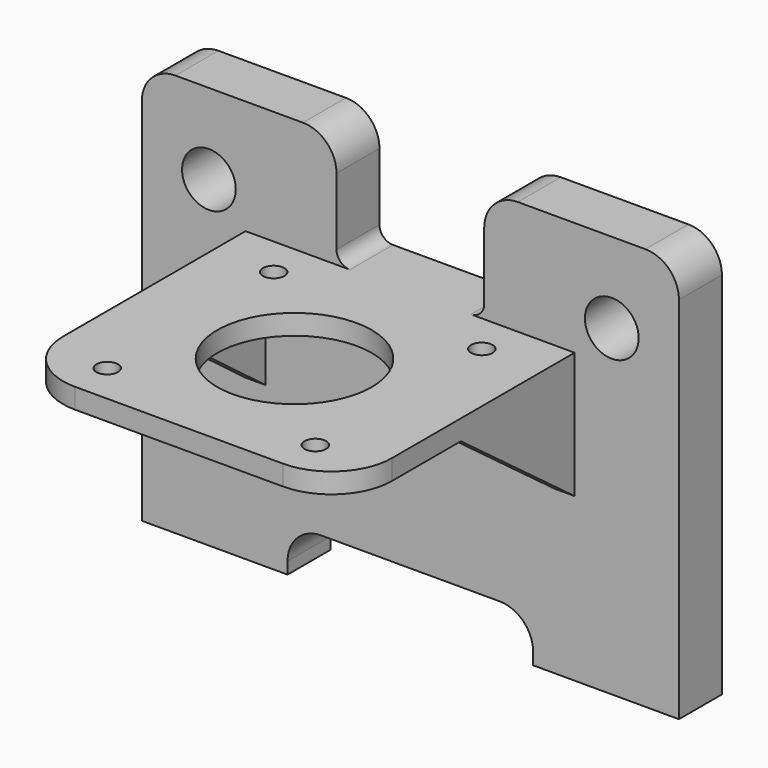
from build123d import *

# Parameters (mm, degrees)
F0_R     = 5
F0_R_2   = 4
F1_DEPTH = 8
F2_W     = 49
F2_H     = 43
F2_R     = 1.6
F2_R_2   = 11.5
F3_DEPTH = 3
F5_DEPTH = 3
F6_R     = 9
F8_DEPTH = 3
F9_DEPTH = 8


# Not quite as in the source:
# - a feature of the source that left no trace in its solid (it failed there, or was rolled back) is left out


with BuildPart() as f1:
    # F0 (on Front) → F1 (new body)
    with BuildSketch(Plane.XZ):
        with BuildLine():
            Line((-15.9509392173, 58.3590910856), (-34.9509392173, 58.3590910856))
            ThreePointArc((-34.9509392173, 58.3590910856), (-38.4864731233, 56.8946249915), (-39.9509392173, 53.3590910856))
            Line((-39.9509392173, 53.3590910856), (-39.9509392173, -1.6409089144))
            Line((-39.9509392173, -1.6409089144), (-18.2393845171, -1.6409089144))
            Line((-18.2393845171, -1.6409089144), (-18.2393845171, 0.1278397727))
            ThreePointArc((-18.2393845171, 0.1278397727), (-16.774918423, 3.6633736787), (-13.2393845171, 5.1278397727))
            Line((-13.2393845171, 5.1278397727), (13.3375060824, 5.1278397727))
            ThreePointArc((13.3375060824, 5.1278397727), (16.8730399883, 3.6633736787), (18.3375060824, 0.1278397727))
            Line((18.3375060824, 0.1278397727), (18.3375060824, -1.6409089144))
            Line((18.3375060824, -1.6409089144), (40.0490607827, -1.6409089144))
            Line((40.0490607827, -1.6409089144), (40.0490607827, 53.3590910856))
            ThreePointArc((40.0490607827, 53.3590910856), (38.5845946886, 56.8946249915), (35.0490607827, 58.3590910856))
            Line((35.0490607827, 58.3590910856), (16.0490607827, 58.3590910856))
            ThreePointArc((16.0490607827, 58.3590910856), (12.5135268767, 56.8946249915), (11.0490607827, 53.3590910856))
            Line((11.0490607827, 53.3590910856), (11.0490607827, 43.3590910856))
            ThreePointArc((11.0490607827, 43.3590910856), (10.463274345, 41.9448775232), (9.0490607827, 41.3590910856))
            Line((9.0490607827, 41.3590910856), (-8.9509392173, 41.3590910856))
            ThreePointArc((-8.9509392173, 41.3590910856), (-10.3651527797, 41.9448775232), (-10.9509392173, 43.3590910856))
            Line((-10.9509392173, 43.3590910856), (-10.9509392173, 53.3590910856))
            ThreePointArc((-10.9509392173, 53.3590910856), (-12.4154053114, 56.8946249915), (-15.9509392173, 58.3590910856))
        make_face()
        with Locations((-29.9509392173, 10.3590910856)):
            Circle(F0_R, mode=Mode.SUBTRACT)
        with Locations((30.0490607827, 10.3590910856)):
            Circle(F0_R, mode=Mode.SUBTRACT)
        with Locations((-29.9509392173, 46.3590910856)):
            Circle(F0_R_2, mode=Mode.SUBTRACT)
        with Locations((30.0490607827, 46.3590910856)):
            Circle(F0_R_2, mode=Mode.SUBTRACT)
    extrude(amount=F1_DEPTH)

    # F2 (on face) → F3 (join)
    with BuildSketch(Plane.XY.offset(41.3590910856)):
        with Locations((0.0111820996, -29.5)):
            Rectangle(F2_W, F2_H)
        with Locations((-15.5, -45)):
            Circle(F2_R, mode=Mode.SUBTRACT)
        with Locations((15.5, -45)):
            Circle(F2_R, mode=Mode.SUBTRACT)
        with Locations((0, -29.5)):
            Circle(F2_R_2, mode=Mode.SUBTRACT)
        with Locations((-15.5, -14)):
            Circle(F2_R, mode=Mode.SUBTRACT)
        with Locations((15.5, -14)):
            Circle(F2_R, mode=Mode.SUBTRACT)
    extrude(amount=-F3_DEPTH)

    # F4 (on face) → F5 (join)
    with BuildSketch(Plane(origin=(-24.4888179004, 0, 0), x_dir=(0, -1, 0), z_dir=(-1, 0, 0))):
        Polygon((29.5, 38.3590910856), (8, 38.3590910856), (7.8833866864, 22.056709975), align=None)
    extrude(amount=-F5_DEPTH)

    # F6
    f6_edges = [f1.edges().sort_by_distance(p)[0] for p in [
        (-24.488818, -51, 39.859091),
        (24.511182, -51, 39.859091),
    ]]
    fillet(f6_edges, radius=F6_R)

    # F7 (on face) → F8 (join)
    with BuildSketch(Plane.YZ.offset(24.5111820996)):
        Polygon((-8, 38.3590910856), (-29.1853044182, 38.3590910856), (-8, 22.5599054247), align=None)
    extrude(amount=-F8_DEPTH)

    # F0 (on Front) → F9 (join)
    with BuildSketch(Plane.XZ):
        with Locations((30.0490607827, 10.3590910856)):
            Circle(F0_R)
        with Locations((-29.9509392173, 10.3590910856)):
            Circle(F0_R)
    extrude(amount=F9_DEPTH)


with BuildPart() as f10_1:
    # F10: copy of F1
    add(f1.part)


solid = f1.part
